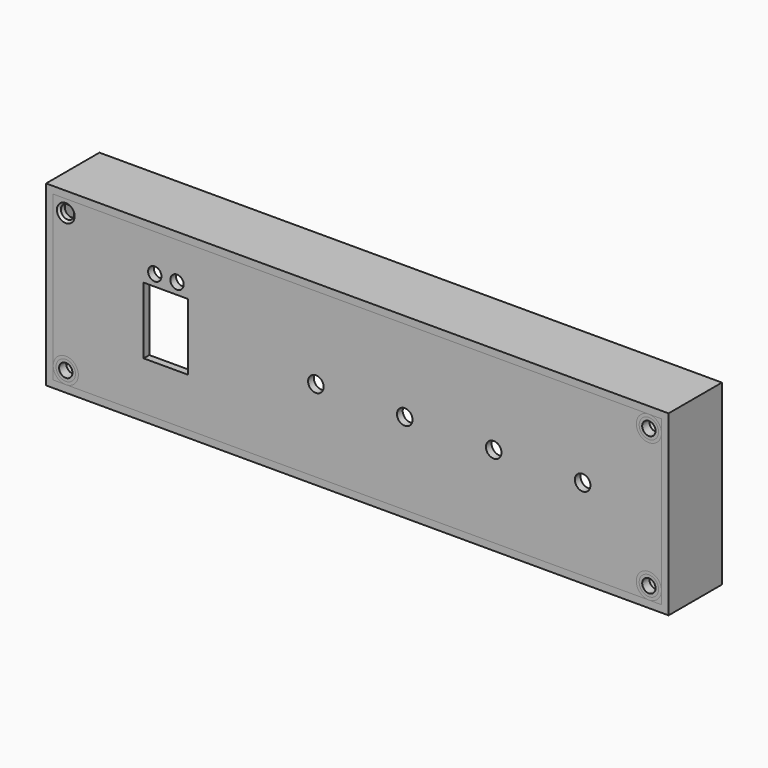
from build123d import *

# Parameters (mm, degrees)
F0_W             = 10
F0_H             = 15
F0_R             = 1.75
F0_R_2           = 1.5
F1_DEPTH         = 1.6
F0_W_2           = 140
F0_H_2           = 40
F2_DEPTH         = 15
F3_DEPTH         = 1.6
F0_R_3           = 2.1826887697
F4_DEPTH         = 6
F4_TAPER         = -3
F0_R_4           = 1.5019252968
F5_DEPTH         = 2
F6_D             = 3
F6_CSINK_D       = 4
F6_CSINK_ANGLE   = 90
F6_2_D           = 3
F6_2_CSINK_D     = 4
F6_2_CSINK_ANGLE = 90


# Not quite as in the source:
# - a feature names something its author has since deleted; it is built from what else it names


with BuildPart() as f1:
    # F0 (on Front) → F1 (new body)
    with BuildSketch(Plane.XZ):
        with BuildLine():
            Line((65.5715732005, 18.4000004083), (-68.4000004083, 18.4000004083))
            Line((-68.4000004083, 18.4000004083), (-68.4000004083, -15.5715732606))
            ThreePointArc((-68.4000004083, -15.5715732606), (-65.5715732721, -12.7431461588), (-62.7431461588, -15.5715732835))
            ThreePointArc((-62.7431461588, -15.5715732835), (-63.5715732835, -17.5715732835), (-65.5715732835, -18.4000004083))
            Line((-65.5715732835, -18.4000004083), (65.5715732835, -18.4000004083))
            ThreePointArc((65.5715732835, -18.4000004083), (63.5715732835, -13.5715732835), (68.4000004083, -15.5715732835))
            Line((68.4000004083, -15.5715732835), (68.4000004083, 15.5715732835))
            ThreePointArc((68.4000004083, 15.5715732835), (63.5715733129, 13.5715732542), (65.5715732005, 18.4000004083))
        make_face()
        with Locations((-43.0512540042, 0)):
            Rectangle(F0_W, F0_H, mode=Mode.SUBTRACT)
        with Locations((-9.3271806836, 0)):
            Circle(F0_R, mode=Mode.SUBTRACT)
        with Locations((-45.5512540042, 10.0292349234)):
            Circle(F0_R_2, mode=Mode.SUBTRACT)
        with Locations((-40.5512540042, 10.0292349234)):
            Circle(F0_R_2, mode=Mode.SUBTRACT)
        with Locations((10.6728193164, 0)):
            Circle(F0_R, mode=Mode.SUBTRACT)
        with Locations((30.6728193164, 0)):
            Circle(F0_R, mode=Mode.SUBTRACT)
        with Locations((50.6728193164, 0)):
            Circle(F0_R, mode=Mode.SUBTRACT)
    extrude(amount=-F1_DEPTH)

    # F6 (through all)
    with Locations(Plane.XZ):
        with Locations((-65.5715732835, 15.5715732835)):
            CounterSinkHole(F6_D / 2, F6_CSINK_D / 2, counter_sink_angle=F6_CSINK_ANGLE)


with BuildPart() as f2:
    # F0 (on Front) → F2 (new body)
    with BuildSketch(Plane.XZ):
        Rectangle(F0_W_2, F0_H_2)
        Polygon((-68.4000004083, -15.5715732606), (-68.4000004083, 18.4000004083), (65.5715732005, 18.4000004083), (68.4000004083, 18.4000004083), (68.4000004083, 15.5715732835), (68.4000004083, -15.5715732835), (68.4000004083, -18.4000004083), (65.5715732835, -18.4000004083), (-65.5715732835, -18.4000004083), (-68.4000004083, -18.4000004083), align=None, mode=Mode.SUBTRACT)
    extrude(amount=-F2_DEPTH)


with BuildPart() as f3:
    # F0 (on Front) → F3 (new body)
    with BuildSketch(Plane.XZ):
        with BuildLine():
            Line((65.5715732005, 18.4000004083), (-68.4000004083, 18.4000004083))
            Line((-68.4000004083, 18.4000004083), (-68.4000004083, -15.5715732606))
            ThreePointArc((-68.4000004083, -15.5715732606), (-65.5715732721, -12.7431461588), (-62.7431461588, -15.5715732835))
            ThreePointArc((-62.7431461588, -15.5715732835), (-63.5715732835, -17.5715732835), (-65.5715732835, -18.4000004083))
            Line((-65.5715732835, -18.4000004083), (65.5715732835, -18.4000004083))
            ThreePointArc((65.5715732835, -18.4000004083), (63.5715732835, -13.5715732835), (68.4000004083, -15.5715732835))
            Line((68.4000004083, -15.5715732835), (68.4000004083, 15.5715732835))
            ThreePointArc((68.4000004083, 15.5715732835), (63.5715733129, 13.5715732542), (65.5715732005, 18.4000004083))
        make_face()
        with Locations((-43.0512540042, 0)):
            Rectangle(F0_W, F0_H, mode=Mode.SUBTRACT)
        with Locations((-9.3271806836, 0)):
            Circle(F0_R, mode=Mode.SUBTRACT)
        with Locations((-45.5512540042, 10.0292349234)):
            Circle(F0_R_2, mode=Mode.SUBTRACT)
        with Locations((-40.5512540042, 10.0292349234)):
            Circle(F0_R_2, mode=Mode.SUBTRACT)
        with Locations((10.6728193164, 0)):
            Circle(F0_R, mode=Mode.SUBTRACT)
        with Locations((30.6728193164, 0)):
            Circle(F0_R, mode=Mode.SUBTRACT)
        with Locations((50.6728193164, 0)):
            Circle(F0_R, mode=Mode.SUBTRACT)
    extrude(amount=-F3_DEPTH)

    # F6#2 (through all)
    with Locations(Plane.XZ):
        with Locations((-65.5715732835, 15.5715732835)):
            CounterSinkHole(F6_2_D / 2, F6_2_CSINK_D / 2, counter_sink_angle=F6_2_CSINK_ANGLE)


with BuildPart() as f3b:
    # F0 (on Front) → F3, piece 2 (new body)
    with BuildSketch(Plane.XZ):
        with BuildLine():
            ThreePointArc((-65.5715732835, -18.4000004083), (-67.5715732917, -17.5715732754), (-68.4000004083, -15.5715732606))
            Line((-68.4000004083, -15.5715732606), (-68.4000004083, -18.4000004083))
            Line((-68.4000004083, -18.4000004083), (-65.5715732835, -18.4000004083))
        make_face()
    extrude(amount=-F3_DEPTH)


with BuildPart() as f3c:
    # F0 (on Front) → F3, piece 3 (new body)
    with BuildSketch(Plane.XZ):
        with BuildLine():
            Line((68.4000004083, -18.4000004083), (68.4000004083, -15.5715732835))
            ThreePointArc((68.4000004083, -15.5715732835), (67.5715732835, -17.5715732835), (65.5715732835, -18.4000004083))
            Line((65.5715732835, -18.4000004083), (68.4000004083, -18.4000004083))
        make_face()
    extrude(amount=-F3_DEPTH)


with BuildPart() as f3d:
    # F0 (on Front) → F3, piece 4 (new body)
    with BuildSketch(Plane.XZ):
        with BuildLine():
            Line((68.4000004083, 18.4000004083), (65.5715732005, 18.4000004083))
            ThreePointArc((65.5715732005, 18.4000004083), (67.5715732542, 17.5715733129), (68.4000004083, 15.5715732835))
            Line((68.4000004083, 15.5715732835), (68.4000004083, 18.4000004083))
        make_face()
    extrude(amount=-F3_DEPTH)


with BuildPart() as f4:
    # F0 (on Front) → F4 (new body)
    with BuildSketch(Plane.XZ):
        with BuildLine():
            ThreePointArc((68.4000004083, 15.5715732835), (67.5715732542, 17.5715733129), (65.5715732005, 18.4000004083))
            ThreePointArc((65.5715732005, 18.4000004083), (63.5715733129, 13.5715732542), (68.4000004083, 15.5715732835))
        make_face()
        with Locations((65.5715732835, 15.5715732835)):
            Circle(F0_R_3, mode=Mode.SUBTRACT)
    extrude(amount=-F4_DEPTH, taper=F4_TAPER)


with BuildPart() as f4b:
    # F0 (on Front) → F4, piece 2 (new body)
    with BuildSketch(Plane.XZ):
        with BuildLine():
            ThreePointArc((65.5715732835, -18.4000004083), (67.5715732835, -17.5715732835), (68.4000004083, -15.5715732835))
            ThreePointArc((68.4000004083, -15.5715732835), (63.5715732835, -13.5715732835), (65.5715732835, -18.4000004083))
        make_face()
        with Locations((65.5715732835, -15.5715732835)):
            Circle(F0_R_3, mode=Mode.SUBTRACT)
    extrude(amount=-F4_DEPTH, taper=F4_TAPER)


with BuildPart() as f4c:
    # F0 (on Front) → F4, piece 3 (new body)
    with BuildSketch(Plane.XZ):
        with BuildLine():
            ThreePointArc((-62.7431461588, -15.5715732835), (-65.5715732721, -12.7431461588), (-68.4000004083, -15.5715732606))
            ThreePointArc((-68.4000004083, -15.5715732606), (-67.5715732917, -17.5715732754), (-65.5715732835, -18.4000004083))
            ThreePointArc((-65.5715732835, -18.4000004083), (-63.5715732835, -17.5715732835), (-62.7431461588, -15.5715732835))
        make_face()
        with Locations((-65.5715732835, -15.5715732835)):
            Circle(F0_R_3, mode=Mode.SUBTRACT)
    extrude(amount=-F4_DEPTH, taper=F4_TAPER)


with BuildPart() as f5:
    # F0 (on Front) → F5 (new body)
    with BuildSketch(Plane.XZ):
        with Locations((65.5715732835, 15.5715732835)):
            Circle(F0_R_3)
        with Locations((65.5715732835, 15.5715732835)):
            Circle(F0_R_4, mode=Mode.SUBTRACT)
    extrude(amount=-F5_DEPTH)


with BuildPart() as f5b:
    # F0 (on Front) → F5, piece 2 (new body)
    with BuildSketch(Plane.XZ):
        with Locations((65.5715732835, -15.5715732835)):
            Circle(F0_R_3)
        with Locations((65.5715732835, -15.5715732835)):
            Circle(F0_R_4, mode=Mode.SUBTRACT)
    extrude(amount=-F5_DEPTH)


with BuildPart() as f5c:
    # F0 (on Front) → F5, piece 3 (new body)
    with BuildSketch(Plane.XZ):
        with Locations((-65.5715732835, -15.5715732835)):
            Circle(F0_R_3)
        with Locations((-65.5715732835, -15.5715732835)):
            Circle(F0_R_4, mode=Mode.SUBTRACT)
    extrude(amount=-F5_DEPTH)


solid = Compound([f1.part, f2.part, f3.part, f3b.part, f3c.part, f3d.part, f4.part, f4b.part, f4c.part, f5.part, f5b.part, f5c.part])
